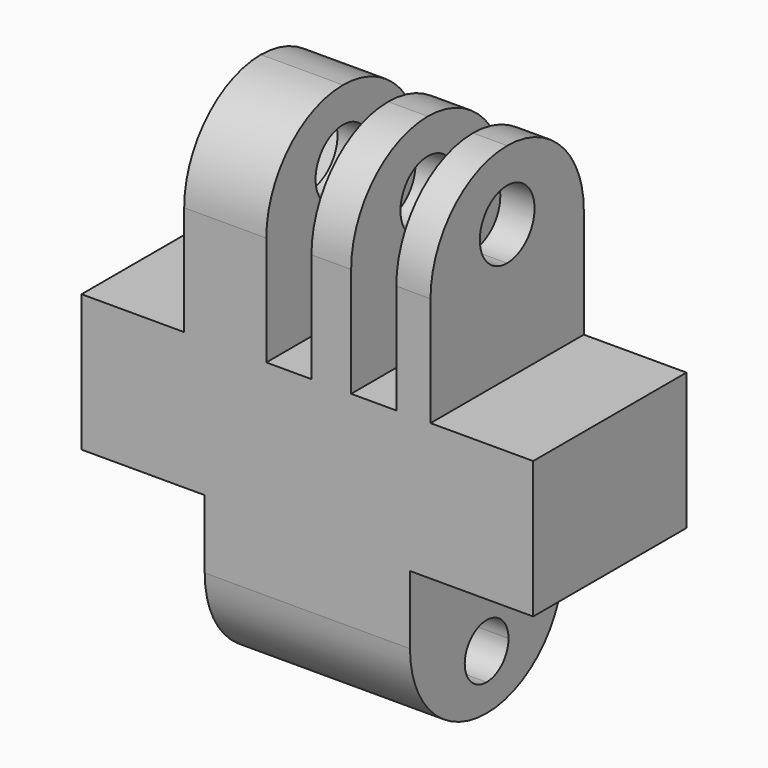
from build123d import *

# Parameters (mm, degrees)
F0_W      = 33
F0_H      = 14
F1_DEPTH  = 10
F2_W      = 15
F2_H      = 14
F3_DEPTH  = 12
F4_R      = 7
F5_R      = 6.99999
F7_DEPTH  = 24.001
F8_W      = 18
F8_H      = 14
F9_DEPTH  = 15
F11_DEPTH = 25
F13_R     = 6.99999
F12_W     = 3.3
F12_H     = 15
F14_DEPTH = 25
F15_R     = 2.5
F16_DEPTH = 3.6


# Not quite as in the source:
# - a fillet or chamfer is up to 0.001 mm smaller than in the source, because OpenCascade refuses the exact size


with BuildPart() as f1:
    # F0 (on Top) → F1 (new body)
    with BuildSketch(Plane.XY):
        with Locations((16.5, -7)):
            Rectangle(F0_W, F0_H)
    extrude(amount=F1_DEPTH)

    # F2 (on face) → F3 (join)
    with BuildSketch(Plane(origin=(0, 0, 0), x_dir=(1, 0, 0), z_dir=(0, 0, -1))):
        with Locations((16.5, 7)):
            Rectangle(F2_W, F2_H)
    extrude(amount=F3_DEPTH)

    # F4
    f4_edges = [f1.edges().sort_by_distance(p)[0] for p in [
        (16.5, 0, -12),
    ]]
    fillet(f4_edges, radius=F4_R)

    # F5 (radius 7 in the source; OpenCascade refuses exactly that, so slightly less here)
    f5_edges = [f1.edges().sort_by_distance(p)[0] for p in [
        (16.5, -14, -12),
    ]]
    fillet(f5_edges, radius=F5_R)

    # F6 (on face) → F7 (cut, through all)
    with BuildSketch(Plane.YZ.offset(24)):
        with BuildLine():
            Line((-7, -10), (-7, -6))
            ThreePointArc((-7, -6), (-9, -8), (-7, -10))
        make_face()
        with BuildLine():
            ThreePointArc((-7, -10), (-5.5857864376, -9.4142135624), (-5, -8))
            ThreePointArc((-5, -8), (-5.5857864376, -6.5857864376), (-7, -6))
            Line((-7, -6), (-7, -10))
        make_face()
    extrude(amount=-F7_DEPTH, mode=Mode.SUBTRACT)

    # F8 (on face) → F9 (join)
    with BuildSketch(Plane.XY.offset(10)):
        with Locations((16.5, -7)):
            Rectangle(F8_W, F8_H)
    extrude(amount=F9_DEPTH)

    # F10 (on face) → F11 (cut)
    with BuildSketch(Plane(origin=(7.5, 0, 0), x_dir=(0, -1, 0), z_dir=(-1, 0, 0))):
        with BuildLine():
            Line((7, 22.4445006251), (7, 17.4445006251))
            ThreePointArc((7, 17.4445006251), (8.767766953, 18.1767336722), (9.5, 19.9445006251))
            ThreePointArc((9.5, 19.9445006251), (8.767766953, 21.7122675781), (7, 22.4445006251))
        make_face()
        with BuildLine():
            ThreePointArc((7, 22.4445006251), (4.5, 19.9445006251), (7, 17.4445006251))
            Line((7, 17.4445006251), (7, 22.4445006251))
        make_face()
    extrude(amount=-F11_DEPTH, mode=Mode.SUBTRACT)

    # F13 (radius 7 in the source; OpenCascade refuses exactly that, so slightly less here)
    f13_edges = [f1.edges().sort_by_distance(p)[0] for p in [
        (16.5, -14, 25),
        (16.5, 0, 25),
    ]]
    fillet(f13_edges, radius=F13_R)

    # F12 (on face) → F14 (cut)
    with BuildSketch(Plane.XZ.offset(14)):
        with Locations((21.35, 17.5)):
            Rectangle(F12_W, F12_H)
        with Locations((15.15, 17.5)):
            Rectangle(F12_W, F12_H)
    extrude(amount=-F14_DEPTH, mode=Mode.SUBTRACT)

    # F15 (on face) → F16 (cut)
    with BuildSketch(Plane(origin=(7.5, 0, 0), x_dir=(0, -1, 0), z_dir=(-1, 0, 0))):
        Polygon((4.7483339502, 16.0445006251), (9.2516660498, 16.0445006251), (11.5033320997, 19.9445006251), (9.2516660498, 23.8445006251), (4.7483339502, 23.8445006251), (2.4966679003, 19.9445006251), align=None)
        with Locations((7, 19.9445006251)):
            Circle(F15_R, mode=Mode.SUBTRACT)
    extrude(amount=-F16_DEPTH, mode=Mode.SUBTRACT)


solid = f1.part
